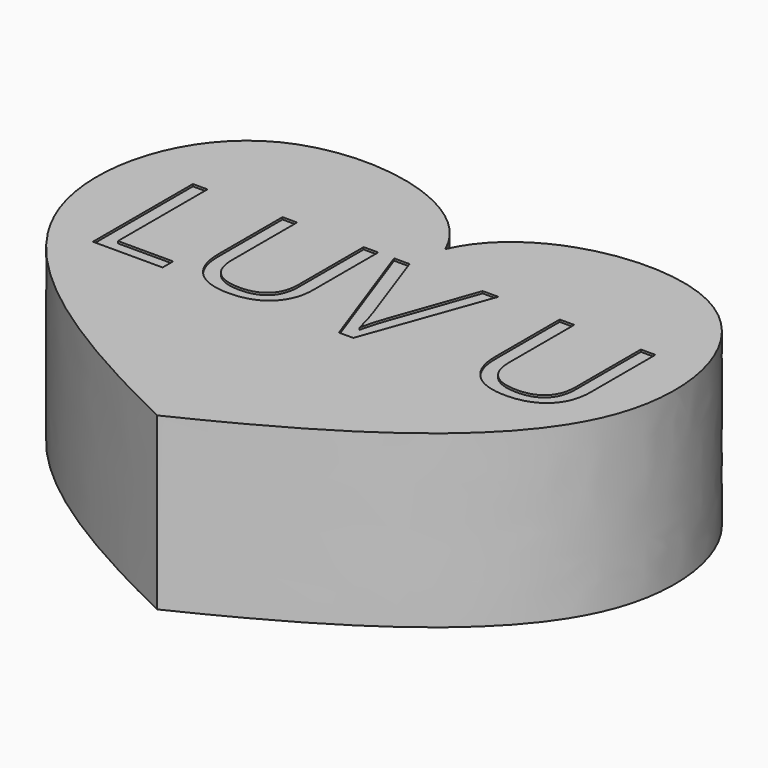
from build123d import *

# Parameters (mm, degrees)
F1_DEPTH     = 20.32
F3_TEXT_SIZE = 20.8338666785
F4_DEPTH     = 0.254


# Not quite as in the source:
# - a feature of the source that left no trace in its solid (it failed there, or was rolled back) is left out
# - Text() gives the source's letters only with a copy of the font that has no kerning and outlines rounded to 1/6400 em; it was checked with that copy


with BuildPart() as f1:
    # F0 (on Top) → F1 (new body)
    with BuildSketch(Plane.XY):
        with BuildLine():
            Line((0, -42.8451001644), (0, 0))
            add(Edge.make_bspline(
                [(0, 0), (-3.6995985123, 8.6103660574), (-30.1452333709, 13.9118496672), (-40.0369162972, -20.4280483879), (-15.6666533057, -35.2612404284), (0, -42.8451001644)],
                knots=[0, 0, 0, 0, 0.3096588007, 0.6039269207, 1, 1, 1, 1], degree=3))
        make_face()
    extrude(amount=F1_DEPTH)

    # F2: F1 across plane


with BuildPart() as f1_1:
    add(f1.part)
    add(f1.part.mirror(Plane.YZ))

    # F3 (on face) → F4 (cut)
    with BuildSketch(Plane.XY.offset(20.32)):
        with Locations((-28.5342591204, -19.2863350124)):
            Text('LUV U', F3_TEXT_SIZE, font='Open Sans', text_align=(TextAlign.LEFT, TextAlign.BOTTOM))
    extrude(amount=-F4_DEPTH, mode=Mode.SUBTRACT)


solid = f1_1.part
